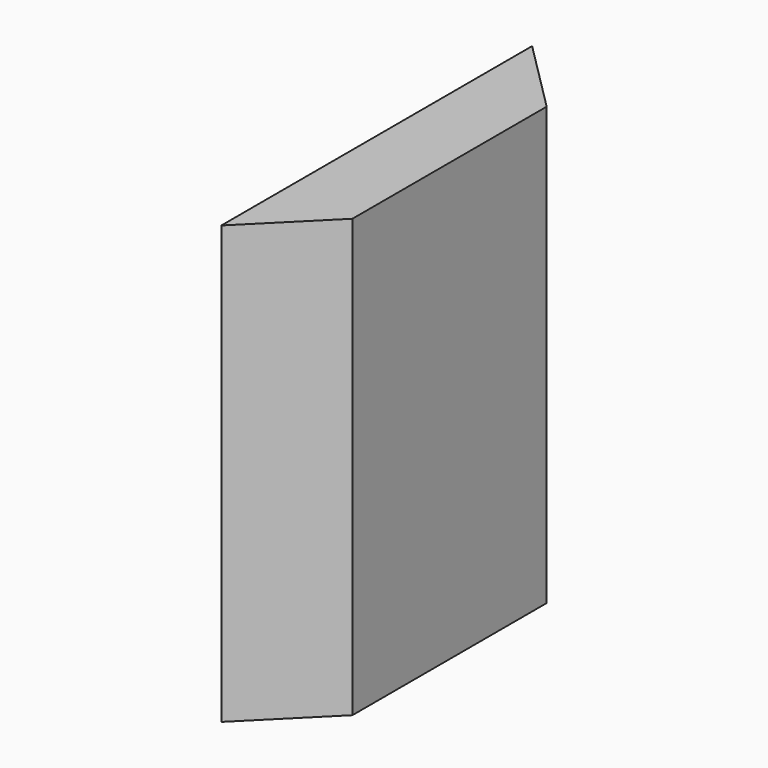
from build123d import *

# Parameters (mm, degrees)
F0_W        = 457.2
F0_H        = 2743.2
F1_DEPTH    = 2743.2
F2_T1_DEPTH = 5878.595898928


# Not quite as in the source:
# - a fillet or chamfer that OpenCascade refuses, or shapes differently, is made with other operations: its cross-section is extruded or revolved along the edge and cut away or added


with BuildPart() as f1:
    # F0 (on Top) → F1 (new body)
    with BuildSketch(Plane.XY):
        with Locations((-125.9096050531, -70.289158705)):
            Rectangle(F0_W, F0_H)
    extrude(amount=F1_DEPTH)

    # F2: chamfer of 609.6 on 2 edges, made by hand

    # F2_s2 → F2_t1 (cut)
    with BuildSketch(Plane.XY.offset(-1567.697949464)):
        Polygon((-506.9096050531, -1441.889158705), (102.6903949469, -832.289158705), (102.6903949469, -1441.889158705), align=None)
        Polygon((102.6903949469, 691.710841295), (-506.9096050531, 1301.310841295), (102.6903949469, 1301.310841295), align=None)
    extrude(amount=F2_T1_DEPTH, mode=Mode.SUBTRACT)


solid = f1.part
